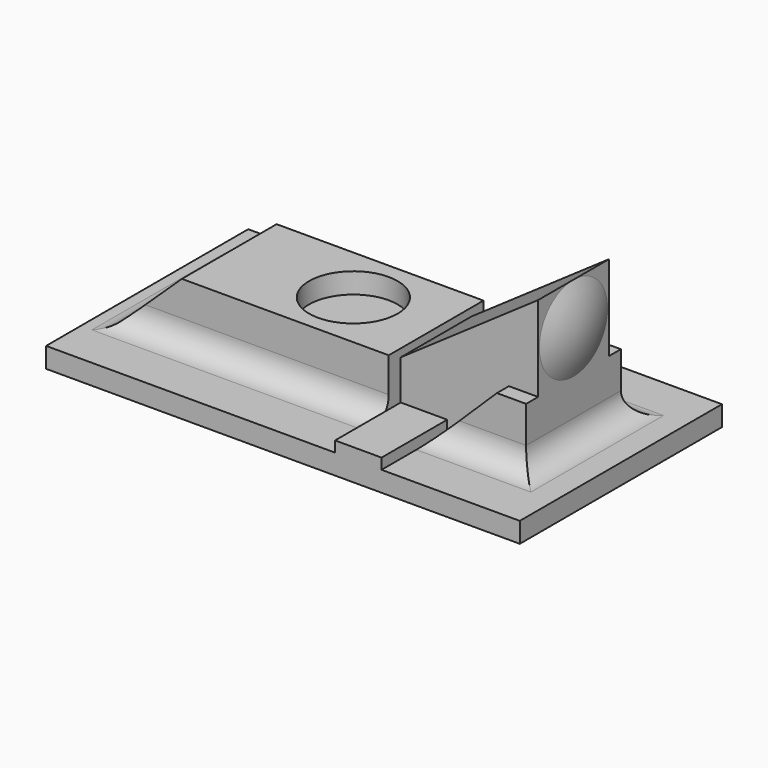
from build123d import *

# Parameters (mm, degrees)
F0_W          = 30
F0_H          = 16
F1_DEPTH      = 1.28
F3_DEPTH      = 3.75
F5_DEPTH      = 2.8
F7_DEPTH      = 3.75
F8_W          = 2.9444776119
F8_H          = 5.2
F9_DEPTH      = 0.68
F10_T1_DEPTH  = 7.5
F10_T6_DEPTH  = 20.75
F10_T11_DEPTH = 24.5
F10_T16_DEPTH = 20.75
F10_T21_DEPTH = 24.5
F10_T26_DEPTH = 9.5055223881
F10_T31_DEPTH = 5.7555223881
F10_T36_DEPTH = 9.5055223881
F10_T41_DEPTH = 5.7555223881
F10_T47_DEPTH = 8.9958162388
F10_T51_DEPTH = 20.75
F10_T59_DEPTH = 20.75
F10_T64_DEPTH = 8.9958162388
F10_T71_DEPTH = 9.5055223881
F10_T76_DEPTH = 11.25
F10_T83_DEPTH = 11.25
F10_T87_DEPTH = 9.5055223881
F11_R         = 2.8
F12_DEPTH     = 1.3
F14_DEPTH     = 2.5


# Not quite as in the source:
# - a fillet or chamfer that OpenCascade refuses, or shapes differently, is made with other operations: its cross-section is extruded or revolved along the edge and cut away or added


with BuildPart() as f1:
    # F0 (on Top) → F1 (new body)
    with BuildSketch(Plane.XY):
        with Locations((1.94, 0)):
            Rectangle(F0_W, F0_H)
    extrude(amount=F1_DEPTH)

    # F2 (on Front) → F3 (join, symmetric)
    with BuildSketch(Plane.XZ):
        Polygon((5.24, 4.98), (-7.86, 4.98), (-11.76, 1.28), (5.24, 1.28), align=None)
    extrude(amount=F3_DEPTH, both=True)

    # F4 (on Front) → F5 (join, symmetric)
    with BuildSketch(Plane.XZ):
        Polygon((13.94, 10.5), (5.24, 4.48), (5.24, -1.6), (12.09, 5.1), (13.94, 5.1), align=None)
    extrude(amount=F5_DEPTH, both=True)

    # F6 (on Front) → F7 (join, symmetric)
    with BuildSketch(Plane.XZ):
        Polygon((13.94, 5.1), (12.09, 5.1), (6.8758208955, 0), (13.94, 0), align=None)
    extrude(amount=F7_DEPTH, both=True)

    # F8 (on face) → F9 (join)
    with BuildSketch(Plane.XY.offset(1.28)):
        with Locations((6.712238806, -5.4)):
            Rectangle(F8_W, F8_H)
        with Locations((6.712238806, 5.4)):
            Rectangle(F8_W, F8_H)
    extrude(amount=F9_DEPTH)

    # F10: fillet of radius 1.5 on 6 edges, made by hand

    # F10_s2 → F10_t1 (join)
    with BuildSketch(Plane.XZ.offset(-3.75)):
        with BuildLine():
            ThreePointArc((15.44, 1.28), (14.3793398282, 1.7193398282), (13.94, 2.78))
            Line((13.94, 2.78), (13.94, 1.28))
            Line((13.94, 1.28), (15.44, 1.28))
        make_face()
        with BuildLine():
            ThreePointArc((-12.3583264955, 1.28), (-11.802580745, 1.3867496058), (-11.3259358476, 1.6918044522))
            Line((-11.3259358476, 1.6918044522), (-11.76, 1.28))
            Line((-11.76, 1.28), (-12.3583264955, 1.28))
        make_face()
    extrude(amount=F10_T1_DEPTH)


with BuildPart() as f10_tool4:
    # F10_s5 → F10_t6 (new body)
    with BuildSketch(Plane.YZ.offset(-15.51)):
        with BuildLine():
            ThreePointArc((-5.25, 1.28), (-4.1893398282, 1.7193398282), (-3.75, 2.78))
            Line((-3.75, 2.78), (-3.75, 1.28))
            Line((-3.75, 1.28), (-5.25, 1.28))
        make_face()
    extrude(amount=F10_T6_DEPTH)

    split(bisect_by=Plane(origin=(-6.2098546713, 0, 6.5455224913), x_dir=(0, 1, 0), z_dir=(0.6882604319, 0, -0.7254636985)), keep=Keep.TOP)


with BuildPart() as f1_1:
    add(f1.part)

    # F10_t3: union F10_tool4
    add(f10_tool4.part)


with BuildPart() as f10_tool9:
    # F10_s10 → F10_t11 (new body)
    with BuildSketch(Plane.YZ.offset(-15.51)):
        with BuildLine():
            ThreePointArc((-5.25, 1.28), (-4.1893398282, 1.7193398282), (-3.75, 2.78))
            Line((-3.75, 2.78), (-3.75, 1.28))
            Line((-3.75, 1.28), (-5.25, 1.28))
        make_face()
    extrude(amount=F10_T11_DEPTH)

    split(bisect_by=Plane(origin=(3.361803676, 0, -3.4370679374), x_dir=(0, 1, 0), z_dir=(0.6992361874, 0, -0.7148907289)), keep=Keep.TOP)


with BuildPart() as f1_2:
    add(f1_1.part)

    # F10_t8: union F10_tool9
    add(f10_tool9.part)


with BuildPart() as f10_tool14:
    # F10_s15 → F10_t16 (new body)
    with BuildSketch(Plane.YZ.offset(-15.51)):
        with BuildLine():
            ThreePointArc((5.25, 1.28), (4.1893398282, 1.7193398282), (3.75, 2.78))
            Line((3.75, 2.78), (3.75, 1.28))
            Line((3.75, 1.28), (5.25, 1.28))
        make_face()
    extrude(amount=F10_T16_DEPTH)

    split(bisect_by=Plane(origin=(-6.2098546713, 0, 6.5455224913), x_dir=(0, 1, 0), z_dir=(0.6882604319, 0, -0.7254636985)), keep=Keep.TOP)


with BuildPart() as f1_3:
    add(f1_2.part)

    # F10_t13: union F10_tool14
    add(f10_tool14.part)


with BuildPart() as f10_tool19:
    # F10_s20 → F10_t21 (new body)
    with BuildSketch(Plane.YZ.offset(-15.51)):
        with BuildLine():
            ThreePointArc((5.25, 1.28), (4.1893398282, 1.7193398282), (3.75, 2.78))
            Line((3.75, 2.78), (3.75, 1.28))
            Line((3.75, 1.28), (5.25, 1.28))
        make_face()
    extrude(amount=F10_T21_DEPTH)

    split(bisect_by=Plane(origin=(3.361803676, 0, -3.4370679374), x_dir=(0, 1, 0), z_dir=(0.6992361874, 0, -0.7148907289)), keep=Keep.TOP)


with BuildPart() as f1_4:
    add(f1_3.part)

    # F10_t18: union F10_tool19
    add(f10_tool19.part)


with BuildPart() as f10_tool24:
    # F10_s25 → F10_t26 (new body)
    with BuildSketch(Plane.YZ.offset(4.4344776119)):
        with BuildLine():
            ThreePointArc((-5.25, 1.28), (-4.1893398282, 1.7193398282), (-3.75, 2.78))
            Line((-3.75, 2.78), (-3.75, 1.28))
            Line((-3.75, 1.28), (-5.25, 1.28))
        make_face()
    extrude(amount=F10_T26_DEPTH)

    split(bisect_by=Plane.YZ.offset(5.24), keep=Keep.BOTTOM)


with BuildPart() as f1_5:
    add(f1_4.part)

    # F10_t23: union F10_tool24
    add(f10_tool24.part)


with BuildPart() as f10_tool29:
    # F10_s30 → F10_t31 (new body)
    with BuildSketch(Plane.YZ.offset(8.1844776119)):
        with BuildLine():
            ThreePointArc((-5.25, 1.28), (-4.1893398282, 1.7193398282), (-3.75, 2.78))
            Line((-3.75, 2.78), (-3.75, 1.28))
            Line((-3.75, 1.28), (-5.25, 1.28))
        make_face()
    extrude(amount=F10_T31_DEPTH)

    split(bisect_by=Plane(origin=(3.361803676, 0, -3.4370679374), x_dir=(0, 1, 0), z_dir=(0.6992361874, 0, -0.7148907289)), keep=Keep.TOP)


with BuildPart() as f1_6:
    add(f1_5.part)

    # F10_t28: union F10_tool29
    add(f10_tool29.part)


with BuildPart() as f10_tool34:
    # F10_s35 → F10_t36 (new body)
    with BuildSketch(Plane.YZ.offset(4.4344776119)):
        with BuildLine():
            ThreePointArc((5.25, 1.28), (4.1893398282, 1.7193398282), (3.75, 2.78))
            Line((3.75, 2.78), (3.75, 1.28))
            Line((3.75, 1.28), (5.25, 1.28))
        make_face()
    extrude(amount=F10_T36_DEPTH)

    split(bisect_by=Plane.YZ.offset(5.24), keep=Keep.BOTTOM)


with BuildPart() as f1_7:
    add(f1_6.part)

    # F10_t33: union F10_tool34
    add(f10_tool34.part)


with BuildPart() as f10_tool39:
    # F10_s40 → F10_t41 (new body)
    with BuildSketch(Plane.YZ.offset(8.1844776119)):
        with BuildLine():
            ThreePointArc((5.25, 1.28), (4.1893398282, 1.7193398282), (3.75, 2.78))
            Line((3.75, 2.78), (3.75, 1.28))
            Line((3.75, 1.28), (5.25, 1.28))
        make_face()
    extrude(amount=F10_T41_DEPTH)

    split(bisect_by=Plane(origin=(3.361803676, 0, -3.4370679374), x_dir=(0, 1, 0), z_dir=(0.6992361874, 0, -0.7148907289)), keep=Keep.TOP)


with BuildPart() as f1_8:
    add(f1_7.part)

    # F10_t38: union F10_tool39
    add(f10_tool39.part)


with BuildPart() as f10_tool45:
    # F10_s46 → F10_t47 (new body)
    with BuildSketch(Plane.XZ.offset(-3.75)):
        with BuildLine():
            ThreePointArc((-12.3583264955, 1.28), (-11.802580745, 1.3867496058), (-11.3259358476, 1.6918044522))
            Line((-11.3259358476, 1.6918044522), (-11.76, 1.28))
            Line((-11.76, 1.28), (-12.3583264955, 1.28))
        make_face()
    extrude(amount=F10_T47_DEPTH)

    split(bisect_by=Plane.XZ.offset(3.75), keep=Keep.TOP)


with BuildPart() as f10_tool49:
    # F10_s50 → F10_t51 (new body)
    with BuildSketch(Plane.YZ.offset(-15.51)):
        with BuildLine():
            ThreePointArc((-5.25, 1.28), (-4.1893398282, 1.7193398282), (-3.75, 2.78))
            Line((-3.75, 2.78), (-3.75, 1.28))
            Line((-3.75, 1.28), (-5.25, 1.28))
        make_face()
    extrude(amount=F10_T51_DEPTH)

    split(bisect_by=Plane.YZ.offset(-13.06), keep=Keep.TOP)

    split(bisect_by=Plane(origin=(-6.2098546713, 0, 6.5455224913), x_dir=(0, 1, 0), z_dir=(-0.6882604319, 0, 0.7254636985)), keep=Keep.TOP)


with BuildPart() as f10_tool45_1:
    add(f10_tool45.part)

    # F10_t54: intersect F10_tool49
    add(f10_tool49.part, mode=Mode.INTERSECT)


with BuildPart() as f1_9:
    add(f1_8.part)

    # F10_t43: union F10_tool45
    add(f10_tool45_1.part)


with BuildPart() as f10_tool57:
    # F10_s58 → F10_t59 (new body)
    with BuildSketch(Plane.YZ.offset(-15.51)):
        with BuildLine():
            ThreePointArc((5.25, 1.28), (4.1893398282, 1.7193398282), (3.75, 2.78))
            Line((3.75, 2.78), (3.75, 1.28))
            Line((3.75, 1.28), (5.25, 1.28))
        make_face()
    extrude(amount=F10_T59_DEPTH)

    split(bisect_by=Plane.YZ.offset(-13.06), keep=Keep.TOP)

    split(bisect_by=Plane(origin=(-6.2098546713, 0, 6.5455224913), x_dir=(0, 1, 0), z_dir=(-0.6882604319, 0, 0.7254636985)), keep=Keep.TOP)


with BuildPart() as f10_tool62:
    # F10_s63 → F10_t64 (new body)
    with BuildSketch(Plane.XZ.offset(-5.2458162388)):
        with BuildLine():
            ThreePointArc((-12.3583264955, 1.28), (-11.802580745, 1.3867496058), (-11.3259358476, 1.6918044522))
            Line((-11.3259358476, 1.6918044522), (-11.76, 1.28))
            Line((-11.76, 1.28), (-12.3583264955, 1.28))
        make_face()
    extrude(amount=F10_T64_DEPTH)

    split(bisect_by=Plane.XZ.offset(-3.75), keep=Keep.BOTTOM)


with BuildPart() as f10_tool57_1:
    add(f10_tool57.part)

    # F10_t66: intersect F10_tool62
    add(f10_tool62.part, mode=Mode.INTERSECT)


with BuildPart() as f1_10:
    add(f1_9.part)

    # F10_t55: union F10_tool57
    add(f10_tool57_1.part)


with BuildPart() as f10_tool69:
    # F10_s70 → F10_t71 (new body)
    with BuildSketch(Plane.YZ.offset(8.1844776119)):
        with BuildLine():
            ThreePointArc((-5.25, 1.28), (-4.1893398282, 1.7193398282), (-3.75, 2.78))
            Line((-3.75, 2.78), (-3.75, 1.28))
            Line((-3.75, 1.28), (-5.25, 1.28))
        make_face()
    extrude(amount=F10_T71_DEPTH)

    split(bisect_by=Plane.YZ.offset(16.94), keep=Keep.BOTTOM)

    split(bisect_by=Plane.YZ.offset(13.94), keep=Keep.TOP)


with BuildPart() as f10_tool74:
    # F10_s75 → F10_t76 (new body)
    with BuildSketch(Plane.XZ.offset(7.5)):
        with BuildLine():
            ThreePointArc((15.44, 1.28), (14.3793398282, 1.7193398282), (13.94, 2.78))
            Line((13.94, 2.78), (13.94, 1.28))
            Line((13.94, 1.28), (15.44, 1.28))
        make_face()
    extrude(amount=-F10_T76_DEPTH)

    split(bisect_by=Plane.XZ.offset(3.75), keep=Keep.TOP)


with BuildPart() as f10_tool69_1:
    add(f10_tool69.part)

    # F10_t78: intersect F10_tool74
    add(f10_tool74.part, mode=Mode.INTERSECT)


with BuildPart() as f1_11:
    add(f1_10.part)

    # F10_t67: union F10_tool69
    add(f10_tool69_1.part)


with BuildPart() as f10_tool81:
    # F10_s82 → F10_t83 (new body)
    with BuildSketch(Plane.XZ.offset(3.75)):
        with BuildLine():
            ThreePointArc((15.44, 1.28), (14.3793398282, 1.7193398282), (13.94, 2.78))
            Line((13.94, 2.78), (13.94, 1.28))
            Line((13.94, 1.28), (15.44, 1.28))
        make_face()
    extrude(amount=-F10_T83_DEPTH)

    split(bisect_by=Plane.XZ.offset(-3.75), keep=Keep.BOTTOM)


with BuildPart() as f10_tool85:
    # F10_s86 → F10_t87 (new body)
    with BuildSketch(Plane.YZ.offset(8.1844776119)):
        with BuildLine():
            ThreePointArc((5.25, 1.28), (4.1893398282, 1.7193398282), (3.75, 2.78))
            Line((3.75, 2.78), (3.75, 1.28))
            Line((3.75, 1.28), (5.25, 1.28))
        make_face()
    extrude(amount=F10_T87_DEPTH)

    split(bisect_by=Plane.YZ.offset(16.94), keep=Keep.BOTTOM)

    split(bisect_by=Plane.YZ.offset(13.94), keep=Keep.TOP)


with BuildPart() as f10_tool81_1:
    add(f10_tool81.part)

    # F10_t90: intersect F10_tool85
    add(f10_tool85.part, mode=Mode.INTERSECT)


with BuildPart() as f1_12:
    add(f1_11.part)

    # F10_t79: union F10_tool81
    add(f10_tool81_1.part)

    # F11 (on face) → F12 (cut)
    with BuildSketch(Plane.XY.offset(4.98)):
        Circle(F11_R)
    extrude(amount=-F12_DEPTH, mode=Mode.SUBTRACT)

    # F13 (on Front) → F14 (cut, symmetric)
    with BuildSketch(Plane.XZ):
        Polygon((-6.56, 3.9), (-10.56, 0), (5.24, 0), (5.24, 3.9), (3.41, 3.9), (1.75, 1.8), (-1.75, 1.8), (-3.41, 3.9), align=None)
        Polygon((11.8855223881, 4.9), (6.8758208955, 0), (13.54, 0), (13.316296041, 4.9), align=None)
    extrude(amount=F14_DEPTH, both=True, mode=Mode.SUBTRACT)

    # F15 (on Front) → F16 (revolve)
    with BuildSketch(Plane.XZ):
        with BuildLine():
            Line((13.94, 7.8), (14.5818286702, 7.8))
            ThreePointArc((14.5818286702, 7.8), (14.4191665899, 9.1876188275), (13.94, 10.5))
            Line((13.94, 10.5), (13.94, 7.8))
        make_face()
    revolve(axis=Axis((14.2609143351, 0, 7.8), (1, 0, 0)))


solid = f1_12.part
